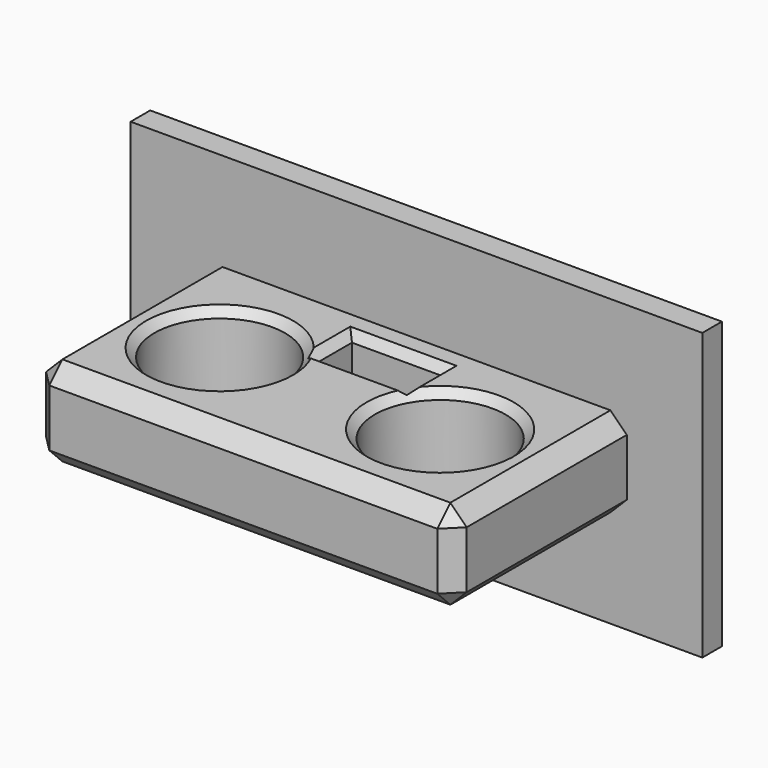
from build123d import *

# Parameters (mm, degrees)
F0_W         = 51.5
F0_H         = 26.5
F0_R         = 8
F1_DEPTH     = 11
F2_W         = 70
F2_H         = 35
F2_W_2       = 25.75
F2_H_2       = 11
F3_DEPTH     = 3
F4_SIZE      = 2
F5_T1_DEPTH  = 11
F5_T3_DEPTH  = 5.5
F5_T17_DEPTH = 8.071682988
F5_T21_DEPTH = 13.571682988
F5_T28_DEPTH = 13.571682988
F5_T32_DEPTH = 8.071682988
F5_T39_DEPTH = 13.571682988
F5_T43_DEPTH = 8.071682988
F5_T50_DEPTH = 13.571682988
F5_T54_DEPTH = 8.071682988
F5_T61_DEPTH = 8.071682988
F5_T65_DEPTH = 13.571682988
F5_T72_DEPTH = 13.571682988
F5_T76_DEPTH = 8.071682988
F5_T83_DEPTH = 13.571682988
F5_T87_DEPTH = 8.071682988
F5_T94_DEPTH = 13.571682988
F5_T98_DEPTH = 8.071682988


# Not quite as in the source:
# - a fillet or chamfer that OpenCascade refuses, or shapes differently, is made with other operations: its cross-section is extruded or revolved along the edge and cut away or added


with BuildPart() as f1:
    # F0 (on Top) → F1 (new body)
    with BuildSketch(Plane.XY):
        Rectangle(F0_W, F0_H)
        Polygon((5.5, 10.25), (22.75, 10.25), (22.75, -10.25), (-22.75, -10.25), (-22.75, 10.25), (-5.5, 10.25), align=None, mode=Mode.SUBTRACT)
        Polygon((22.75, -10.25), (22.75, 10.25), (5.5, 10.25), (5.5, 4.75), (-5.5, 4.75), (-5.5, 10.25), (-22.75, 10.25), (-22.75, -10.25), align=None)
        with Locations((-13.5, 0)):
            Circle(F0_R, mode=Mode.SUBTRACT)
        with BuildLine():
            ThreePointArc((21.5, 0), (13.5, -8), (5.5, 0))
            ThreePointArc((5.5, 0), (13.5, 8), (21.5, 0))
        make_face(mode=Mode.SUBTRACT)
    extrude(amount=F1_DEPTH)

    # F2 (on face) → F3 (join)
    with BuildSketch(Plane(origin=(0, 13.25, 0), x_dir=(-1, 0, 0), z_dir=(0, 1, 0))):
        with Locations((0, 5.5)):
            Rectangle(F2_W, F2_H)
        Polygon((25.75, 0), (0, 0), (-25.75, 0), (-25.75, 11), (0, 11), (25.75, 11), align=None, mode=Mode.SUBTRACT)
        with Locations((-12.875, 5.5)):
            Rectangle(F2_W_2, F2_H_2)
        with Locations((12.875, 5.5)):
            Rectangle(F2_W_2, F2_H_2)
    extrude(amount=F3_DEPTH)

    # F4
    f4_edges = [f1.edges().sort_by_distance(p)[0] for p in [
        (-25.75, -13.25, 5.5),
        (25.75, -13.25, 5.5),
        (0, -13.25, 11),
        (25.75, 0, 11),
        (-25.75, 0, 11),
        (25.75, 0, 0),
        (-25.75, 0, 0),
        (0, -13.25, 0),
    ]]
    chamfer(f4_edges, length=F4_SIZE)

    # F5: chamfer of 1 on 12 edges, made by hand

    # F5_s2 → F5_t1 (cut)
    with BuildSketch(Plane.YZ.offset(-5.5)):
        Polygon((3.75, 0), (4.75, 1), (4.75, 0), align=None)
        Polygon((11.25, 0), (10.25, 1), (10.25, 0), align=None)
        Polygon((3.75, 11), (4.75, 10), (4.75, 11), align=None)
        Polygon((11.25, 11), (10.25, 10), (10.25, 11), align=None)
    extrude(amount=F5_T1_DEPTH, mode=Mode.SUBTRACT)

    # F5_s4 → F5_t3 (cut)
    with BuildSketch(Plane.XZ.offset(-10.25)):
        Polygon((6.5, 0), (5.5, 1), (5.5, 0), align=None)
        Polygon((-6.5, 0), (-5.5, 1), (-5.5, 0), align=None)
        Polygon((-6.5, 11), (-5.5, 10), (-5.5, 11), align=None)
        Polygon((6.5, 11), (5.5, 10), (5.5, 11), align=None)
    extrude(amount=F5_T3_DEPTH, mode=Mode.SUBTRACT)

    # F5_s5 → F5_t6 (revolve, cut)
    with BuildSketch(Plane.XZ):
        Polygon((-4.5, 0), (-5.5, 1), (-5.5, 0), align=None)
    revolve(axis=Axis((-13.5, 0, 0), (0, 0, 1)), mode=Mode.SUBTRACT)

    # F5_s7 → F5_t8 (revolve, cut)
    with BuildSketch(Plane.XZ):
        Polygon((4.5, 0), (5.5, 1), (5.5, 0), align=None)
    revolve(axis=Axis((13.5, 0, 0), (0, 0, -1)), mode=Mode.SUBTRACT)

    # F5_s9 → F5_t10 (revolve, cut)
    with BuildSketch(Plane.XZ):
        Polygon((-4.5, 11), (-5.5, 10), (-5.5, 11), align=None)
    revolve(axis=Axis((-13.5, 0, 11), (0, 0, 1)), mode=Mode.SUBTRACT)

    # F5_s11 → F5_t12 (revolve, cut)
    with BuildSketch(Plane.XZ):
        Polygon((4.5, 11), (5.5, 10), (5.5, 11), align=None)
    revolve(axis=Axis((13.5, 0, 11), (0, 0, -1)), mode=Mode.SUBTRACT)


with BuildPart() as f5_tool15:
    # F5_s16 → F5_t17 (new body)
    with BuildSketch(Plane.XZ.offset(-10.25)):
        Polygon((6.5, 0), (5.5, 1), (5.5, 0), align=None)
    extrude(amount=F5_T17_DEPTH)

    split(bisect_by=Plane.XZ.offset(-4.75), keep=Keep.TOP)


with BuildPart() as f5_tool19:
    # F5_s20 → F5_t21 (new body)
    with BuildSketch(Plane.YZ.offset(8.071682988)):
        Polygon((3.75, 0), (4.75, 1), (4.75, 0), align=None)
    extrude(amount=-F5_T21_DEPTH)

    split(bisect_by=Plane.YZ.offset(5.5), keep=Keep.TOP)


with BuildPart() as f5_tool15_1:
    add(f5_tool15.part)

    # F5_t23: intersect F5_tool19
    add(f5_tool19.part, mode=Mode.INTERSECT)


with BuildPart() as f1_1:
    add(f1.part)

    # F5_t13: cut F5_tool15
    add(f5_tool15_1.part, mode=Mode.SUBTRACT)


with BuildPart() as f5_tool26:
    # F5_s27 → F5_t28 (new body)
    with BuildSketch(Plane.YZ.offset(5.5)):
        Polygon((3.75, 0), (4.75, 1), (4.75, 0), align=None)
    extrude(amount=-F5_T28_DEPTH)

    split(bisect_by=Plane.YZ.offset(-5.5), keep=Keep.BOTTOM)


with BuildPart() as f5_tool30:
    # F5_s31 → F5_t32 (new body)
    with BuildSketch(Plane.XZ.offset(-2.178317012)):
        Polygon((-6.5, 0), (-5.5, 1), (-5.5, 0), align=None)
    extrude(amount=-F5_T32_DEPTH)

    split(bisect_by=Plane.XZ.offset(-4.75), keep=Keep.TOP)


with BuildPart() as f5_tool26_1:
    add(f5_tool26.part)

    # F5_t34: intersect F5_tool30
    add(f5_tool30.part, mode=Mode.INTERSECT)


with BuildPart() as f1_2:
    add(f1_1.part)

    # F5_t24: cut F5_tool26
    add(f5_tool26_1.part, mode=Mode.SUBTRACT)


with BuildPart() as f5_tool37:
    # F5_s38 → F5_t39 (new body)
    with BuildSketch(Plane.YZ.offset(-5.5)):
        Polygon((11.25, 0), (10.25, 1), (10.25, 0), align=None)
    extrude(amount=F5_T39_DEPTH)

    split(bisect_by=Plane.YZ.offset(5.5), keep=Keep.TOP)


with BuildPart() as f5_tool41:
    # F5_s42 → F5_t43 (new body)
    with BuildSketch(Plane.XZ.offset(-12.821682988)):
        Polygon((6.5, 0), (5.5, 1), (5.5, 0), align=None)
    extrude(amount=F5_T43_DEPTH)

    split(bisect_by=Plane.XZ.offset(-10.25), keep=Keep.BOTTOM)


with BuildPart() as f5_tool37_1:
    add(f5_tool37.part)

    # F5_t45: intersect F5_tool41
    add(f5_tool41.part, mode=Mode.INTERSECT)


with BuildPart() as f1_3:
    add(f1_2.part)

    # F5_t35: cut F5_tool37
    add(f5_tool37_1.part, mode=Mode.SUBTRACT)


with BuildPart() as f5_tool48:
    # F5_s49 → F5_t50 (new body)
    with BuildSketch(Plane.YZ.offset(-8.071682988)):
        Polygon((11.25, 0), (10.25, 1), (10.25, 0), align=None)
    extrude(amount=F5_T50_DEPTH)

    split(bisect_by=Plane.YZ.offset(-5.5), keep=Keep.BOTTOM)


with BuildPart() as f5_tool52:
    # F5_s53 → F5_t54 (new body)
    with BuildSketch(Plane.XZ.offset(-4.75)):
        Polygon((-6.5, 0), (-5.5, 1), (-5.5, 0), align=None)
    extrude(amount=-F5_T54_DEPTH)

    split(bisect_by=Plane.XZ.offset(-10.25), keep=Keep.BOTTOM)


with BuildPart() as f5_tool48_1:
    add(f5_tool48.part)

    # F5_t56: intersect F5_tool52
    add(f5_tool52.part, mode=Mode.INTERSECT)


with BuildPart() as f1_4:
    add(f1_3.part)

    # F5_t46: cut F5_tool48
    add(f5_tool48_1.part, mode=Mode.SUBTRACT)


with BuildPart() as f5_tool59:
    # F5_s60 → F5_t61 (new body)
    with BuildSketch(Plane.XZ.offset(-10.25)):
        Polygon((6.5, 11), (5.5, 10), (5.5, 11), align=None)
    extrude(amount=F5_T61_DEPTH)

    split(bisect_by=Plane.XZ.offset(-4.75), keep=Keep.TOP)


with BuildPart() as f5_tool63:
    # F5_s64 → F5_t65 (new body)
    with BuildSketch(Plane.YZ.offset(8.071682988)):
        Polygon((3.75, 11), (4.75, 10), (4.75, 11), align=None)
    extrude(amount=-F5_T65_DEPTH)

    split(bisect_by=Plane.YZ.offset(5.5), keep=Keep.TOP)


with BuildPart() as f5_tool59_1:
    add(f5_tool59.part)

    # F5_t67: intersect F5_tool63
    add(f5_tool63.part, mode=Mode.INTERSECT)


with BuildPart() as f1_5:
    add(f1_4.part)

    # F5_t57: cut F5_tool59
    add(f5_tool59_1.part, mode=Mode.SUBTRACT)


with BuildPart() as f5_tool70:
    # F5_s71 → F5_t72 (new body)
    with BuildSketch(Plane.YZ.offset(5.5)):
        Polygon((3.75, 11), (4.75, 10), (4.75, 11), align=None)
    extrude(amount=-F5_T72_DEPTH)

    split(bisect_by=Plane.YZ.offset(-5.5), keep=Keep.BOTTOM)


with BuildPart() as f5_tool74:
    # F5_s75 → F5_t76 (new body)
    with BuildSketch(Plane.XZ.offset(-2.178317012)):
        Polygon((-6.5, 11), (-5.5, 10), (-5.5, 11), align=None)
    extrude(amount=-F5_T76_DEPTH)

    split(bisect_by=Plane.XZ.offset(-4.75), keep=Keep.TOP)


with BuildPart() as f5_tool70_1:
    add(f5_tool70.part)

    # F5_t78: intersect F5_tool74
    add(f5_tool74.part, mode=Mode.INTERSECT)


with BuildPart() as f1_6:
    add(f1_5.part)

    # F5_t68: cut F5_tool70
    add(f5_tool70_1.part, mode=Mode.SUBTRACT)


with BuildPart() as f5_tool81:
    # F5_s82 → F5_t83 (new body)
    with BuildSketch(Plane.YZ.offset(-8.071682988)):
        Polygon((11.25, 11), (10.25, 10), (10.25, 11), align=None)
    extrude(amount=F5_T83_DEPTH)

    split(bisect_by=Plane.YZ.offset(-5.5), keep=Keep.BOTTOM)


with BuildPart() as f5_tool85:
    # F5_s86 → F5_t87 (new body)
    with BuildSketch(Plane.XZ.offset(-4.75)):
        Polygon((-6.5, 11), (-5.5, 10), (-5.5, 11), align=None)
    extrude(amount=-F5_T87_DEPTH)

    split(bisect_by=Plane.XZ.offset(-10.25), keep=Keep.BOTTOM)


with BuildPart() as f5_tool81_1:
    add(f5_tool81.part)

    # F5_t89: intersect F5_tool85
    add(f5_tool85.part, mode=Mode.INTERSECT)


with BuildPart() as f1_7:
    add(f1_6.part)

    # F5_t79: cut F5_tool81
    add(f5_tool81_1.part, mode=Mode.SUBTRACT)


with BuildPart() as f5_tool92:
    # F5_s93 → F5_t94 (new body)
    with BuildSketch(Plane.YZ.offset(-5.5)):
        Polygon((11.25, 11), (10.25, 10), (10.25, 11), align=None)
    extrude(amount=F5_T94_DEPTH)

    split(bisect_by=Plane.YZ.offset(5.5), keep=Keep.TOP)


with BuildPart() as f5_tool96:
    # F5_s97 → F5_t98 (new body)
    with BuildSketch(Plane.XZ.offset(-12.821682988)):
        Polygon((6.5, 11), (5.5, 10), (5.5, 11), align=None)
    extrude(amount=F5_T98_DEPTH)

    split(bisect_by=Plane.XZ.offset(-10.25), keep=Keep.BOTTOM)


with BuildPart() as f5_tool92_1:
    add(f5_tool92.part)

    # F5_t100: intersect F5_tool96
    add(f5_tool96.part, mode=Mode.INTERSECT)


with BuildPart() as f1_8:
    add(f1_7.part)

    # F5_t90: cut F5_tool92
    add(f5_tool92_1.part, mode=Mode.SUBTRACT)


solid = f1_8.part
